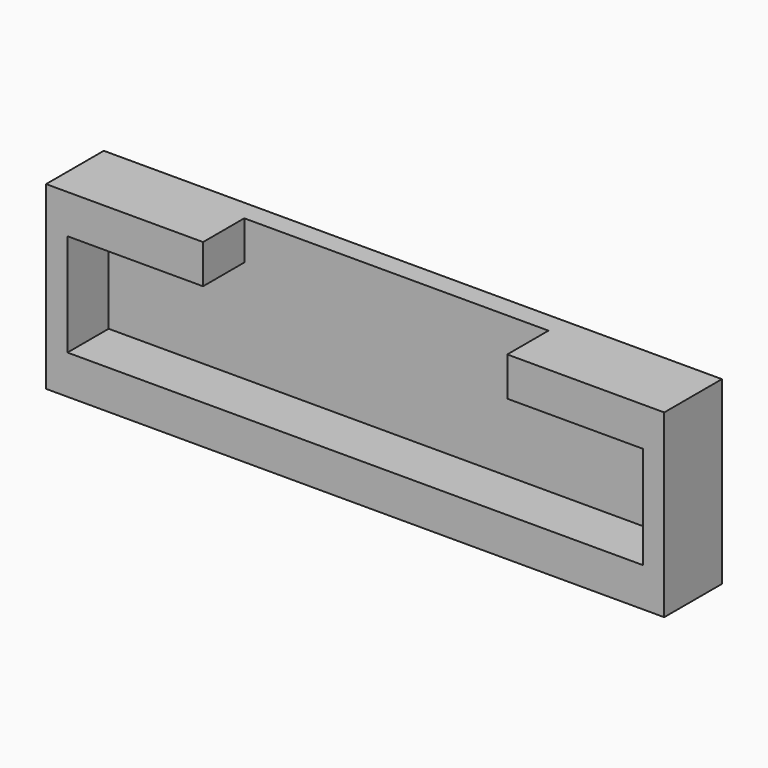
from build123d import *

# Parameters (mm, degrees)
F0_W     = 304.8
F0_H     = 88.9
F1_DEPTH = 35.56
F3_DEPTH = 25.4
F4_DEPTH = 25.4
F2_W     = 66.8579302463
F2_H     = 50.5015006546
F2_W_2   = 66.8579153451
F5_DEPTH = 25.4


# Not quite as in the source:
# - a feature names something its author has since deleted; it is built from what else it names


with BuildPart() as f1:
    # F0 (on Front) → F1 (new body)
    with BuildSketch(Plane.XZ):
        Rectangle(F0_W, F0_H)
    extrude(amount=F1_DEPTH)

    # F2 (on face) → F3 (cut)
    with BuildSketch(Plane.XZ.offset(35.56)):
        Polygon((-33.3375, 19.1518365622), (-33.3375, 44.45), (-74.9989692254, 44.45), (-74.9989692254, 25.2507503273), (-74.9989692254, -25.2507503273), (74.9989692254, -25.2507503273), (74.9989692254, 25.2507503273), (74.9989692254, 44.45), (33.3375, 44.45), (33.3375, 19.1518365622), align=None)
    extrude(amount=-F3_DEPTH, mode=Mode.SUBTRACT)

    # F4 (cut): a face of the model
    f4_faces = [f1.faces().sort_by_distance(p)[0] for p in [
        (0, -35.56, 31.8009182811),
    ]]
    extrude(f4_faces, amount=-F4_DEPTH, mode=Mode.SUBTRACT)

    # F2 (on face) → F5 (cut)
    with BuildSketch(Plane.XZ.offset(35.56)):
        with Locations((-108.4279343486, 0)):
            Rectangle(F2_W, F2_H)
        with Locations((108.427926898, 0)):
            Rectangle(F2_W_2, F2_H)
    extrude(amount=-F5_DEPTH, mode=Mode.SUBTRACT)


solid = f1.part
